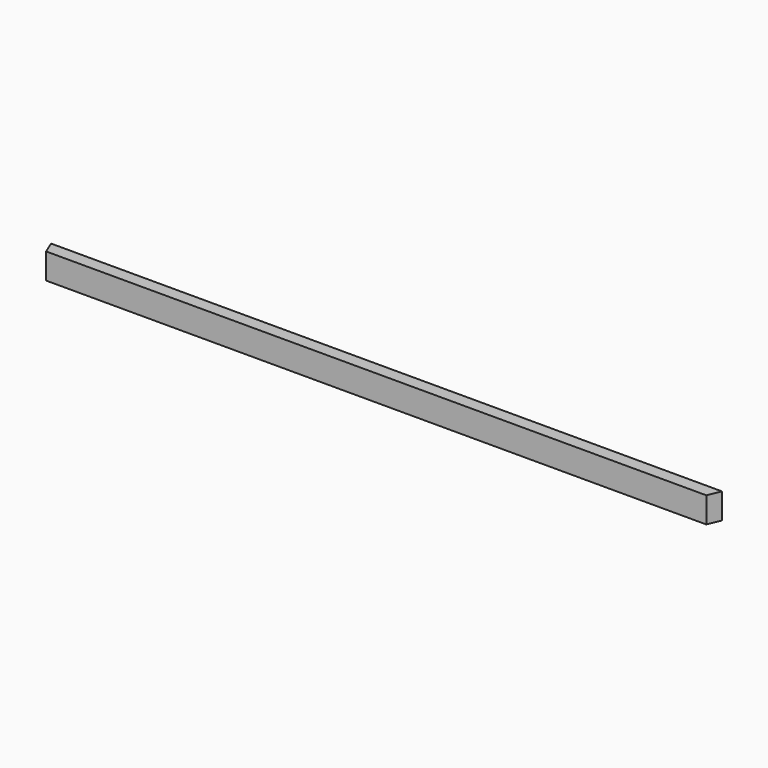
from build123d import *

# Parameters (mm, degrees)
F0_W     = 2654.3
F0_H     = 101.6
F1_DEPTH = 50.8
F3_DEPTH = 163.068


# Not quite as in the source:
# - a feature names something its author has since deleted; it is built from what else it names


with BuildPart() as f1:
    # F0 (on Front) → F1 (new body)
    with BuildSketch(Plane.XZ):
        with Locations((13.1655312276, -1028.2636712667)):
            Rectangle(F0_W, F0_H)
    extrude(amount=F1_DEPTH)

    # F2 (on face) → F3 (cut)
    with BuildSketch(Plane(origin=(0, 0, -1079.0636712667), x_dir=(1, 0, 0), z_dir=(0, 0, -1))):
        Polygon((-1292.9424198039, 50.8), (-1313.9844687724, 50.8), (-1313.9844687724, 0), align=None)
        Polygon((1340.3155312276, 0), (1340.3155312276, 50.8), (1319.273482259, 50.8), align=None)
    extrude(amount=-F3_DEPTH, mode=Mode.SUBTRACT)


solid = f1.part
